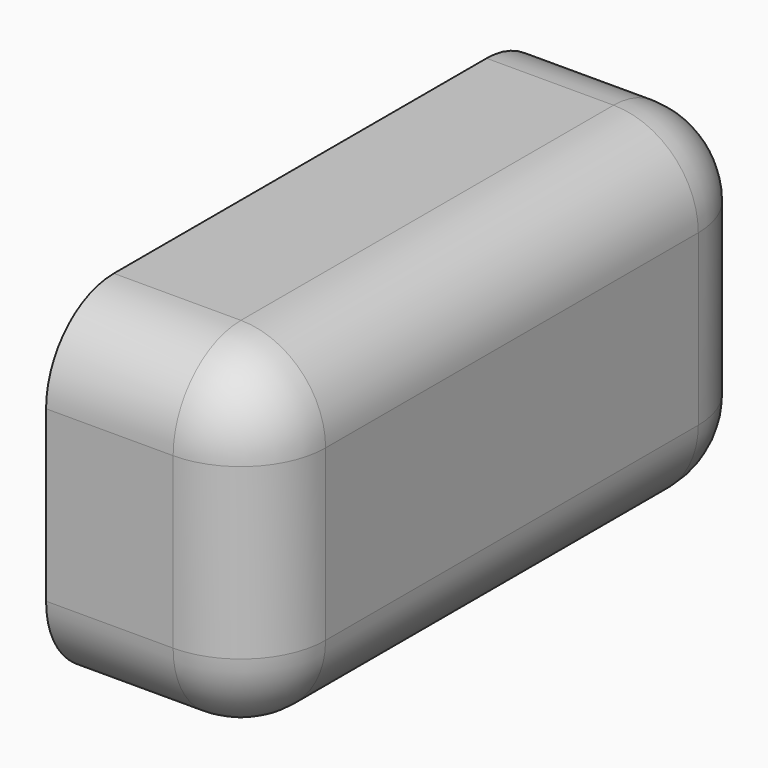
from build123d import *

# Parameters (mm, degrees)
F0_W     = 15
F0_H     = 8
F1_DEPTH = 2.5
F2_T     = -1.25
F3_R     = 2


# Not quite as in the source:
# - a feature names something its author has since deleted; it is built from what else it names


with BuildPart() as f1:
    # F0 (on Right) → F1 (new body, symmetric)
    with BuildSketch(Plane.YZ):
        Rectangle(F0_W, F0_H)
    extrude(amount=F1_DEPTH, both=True)

    # F2
    f2_openings = [f1.faces().sort_by_distance(p)[0] for p in [
        (-2.5, 0, 0),
    ]]
    offset(amount=F2_T, openings=f2_openings)

    # F3
    f3_edges = [f1.edges().sort_by_distance(p)[0] for p in [
        (2.5, 0, 4),
        (2.5, -7.5, 0),
        (2.5, 0, -4),
        (2.5, 7.5, 0),
        (0, -7.5, 4),
        (0, 7.5, 4),
        (0, 7.5, -4),
        (0, -7.5, -4),
    ]]
    fillet(f3_edges, radius=F3_R)


solid = f1.part
